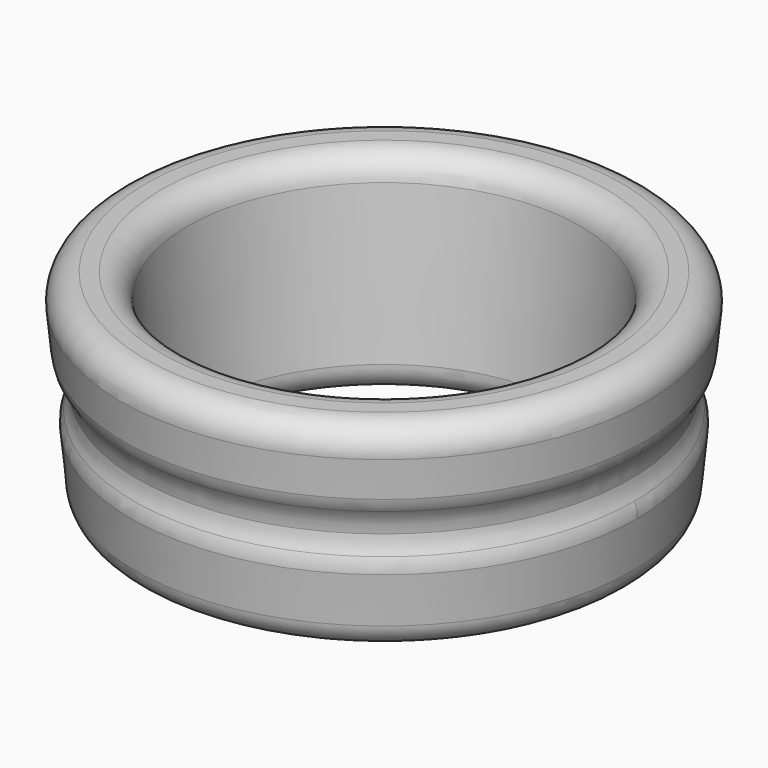
from build123d import *

# Parameters (mm, degrees)
F1_R  = 1.5
F5_R  = 9.55
F6_R  = 10.35
F8_R  = 7.7
F9_R  = 7.15
F12_R = 1


with BuildPart() as f2:
    # F1 (on Front) → F2 (revolve)
    with BuildSketch(Plane.XZ):
        with Locations((-11.05, 0)):
            Circle(F1_R)
    revolve(axis=Axis((0, 0, 0), (0, 0, 1)))


with BuildPart() as f7:
    # F5 (on offset) → F7 section 0
    with BuildSketch(Plane.XY.offset(-4)):
        Circle(F5_R)
    # F6 (on offset) → F7 section 1
    with BuildSketch(Plane.XY.offset(4)):
        Circle(F6_R)
    loft()

    # F8 (on face) → F10 section 0
    with BuildSketch(Plane.XY.offset(4)):
        Circle(F8_R)
    # F9 (on face) → F10 section 1
    with BuildSketch(Plane.XY.offset(-4)):
        Circle(F9_R)
    loft(mode=Mode.SUBTRACT)

    # F11: cut F2
    add(f2.part, mode=Mode.SUBTRACT)

    # F12
    f12_edges = [f7.edges().sort_by_distance(p)[0] for p in [
        (-7.7, 0, 4),
        (-10.35, 0, 4),
        (9.55, 0, 0),
        (-9.55, 0, -4),
        (-7.15, 0, -4),
        (0, 9.858834, -0.91166),
        (0, -9.858834, -0.91166),
        (0, -10.062948, 1.129482),
        (0, 10.062948, 1.129482),
    ]]
    fillet(f12_edges, radius=F12_R)


solid = f7.part
